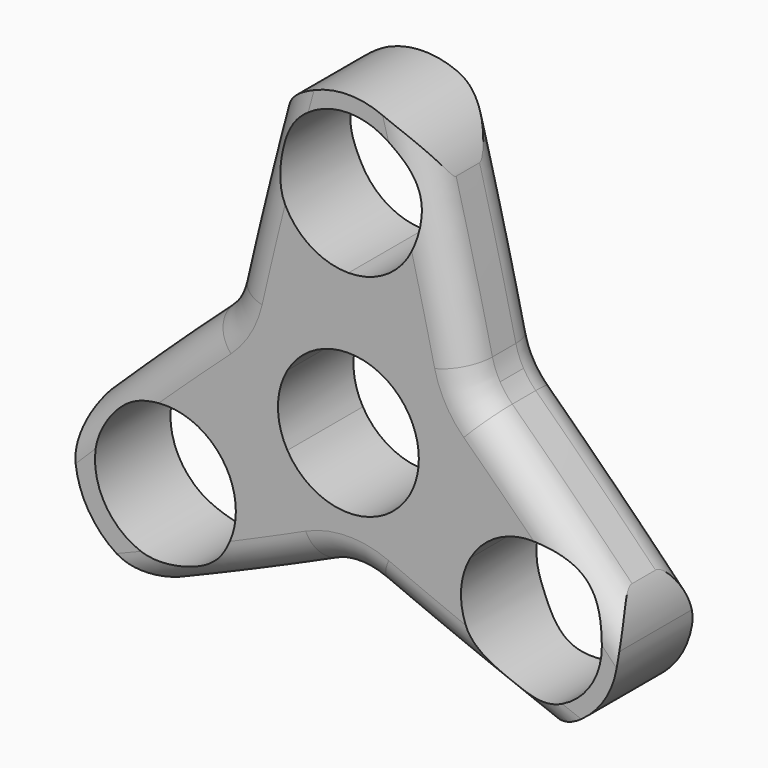
from build123d import *

# Parameters (mm, degrees)
F1_DEPTH     = 14.732
F2_T1_DEPTH  = 93.1608998229
F2_T3_DEPTH  = 105.6007192325
F2_T5_DEPTH  = 102.6342510382
F2_T7_DEPTH  = 101.1360229165
F2_T9_DEPTH  = 92.8404275057
F2_T11_DEPTH = 101.5905654736
F3_T3_ANGLE  = 47.4760223414
F3_T6_ANGLE  = 33.2408882111
F3_T9_ANGLE  = 34.8968457707
F3_T12_ANGLE = 2.7372148443
F3_T15_ANGLE = 2.8789593755
F3_T18_ANGLE = 2.9381084854
F3_T21_ANGLE = 2.7373414603
F3_T24_ANGLE = 2.9000589004
F3_T27_ANGLE = 2.9243217111
F4_T2_ANGLE  = 34.8968457707
F4_T4_ANGLE  = 33.2408882111
F4_T6_ANGLE  = 47.4760223414
F4_T8_ANGLE  = 2.9243217111
F4_T10_ANGLE = 2.9000589004
F4_T12_ANGLE = 2.8789593755
F4_T14_ANGLE = 2.7372148443
F4_T16_ANGLE = 2.7373414603
F4_T18_ANGLE = 2.9381084854


# Not quite as in the source:
# - a fillet or chamfer that OpenCascade refuses, or shapes differently, is made with other operations: its cross-section is extruded or revolved along the edge and cut away or added


with BuildPart() as f1:
    # F0 (on Front) → F1 (new body)
    with BuildSketch(Plane.XZ):
        with BuildLine():
            ThreePointArc((9.5262794416, 5.5), (10.6251840892, 2.8470094961), (11, 0))
            ThreePointArc((11, 0), (10.6251840892, -2.8470094961), (9.5262794416, -5.5))
            Line((9.5262794416, -5.5), (16.8874953738, -9.75))
            ThreePointArc((16.8874953738, -9.75), (28.5479373043, -3.0000353657), (40.239157826, -9.6965487338))
            Line((40.239157826, -9.6965487338), (31.0803296346, 6.00061125))
            ThreePointArc((31.0803296346, 6.00061125), (24.510706985, 6.8563515201), (19.6241089469, 11.3299845831))
            Line((19.6241089469, 11.3299845831), (9.5262794416, 5.5))
        make_face()
        with BuildLine():
            ThreePointArc((0, 11), (5.5, 9.5262794416), (9.5262794416, 5.5))
            Line((9.5262794416, 5.5), (19.6241089469, 11.3299845831))
            ThreePointArc((19.6241089469, 11.3299845831), (18.1888081178, 17.7485475745), (20.6723210956, 23.8387202021))
            Line((20.6723210956, 23.8387202021), (12.7673255725, 37.3869576844))
            ThreePointArc((12.7673255725, 37.3869576844), (13.3155716218, 35.2238597945), (13.5, 33))
            ThreePointArc((13.5, 33), (9.545941546, 23.454058454), (0, 19.5))
            Line((0, 19.5), (0, 11))
        make_face()
        with BuildLine():
            Line((16.8874953738, -9.75), (9.5262794416, -5.5))
            ThreePointArc((9.5262794416, -5.5), (0, -11), (-9.5262794416, -5.5))
            Line((-9.5262794416, -5.5), (-16.3617556921, -9.4464640532))
            ThreePointArc((-16.3617556921, -9.4464640532), (-14.9524532496, -12.8488211233), (-14.4717664314, -16.5))
            ThreePointArc((-14.4717664314, -16.5), (-18.4982539824, -26.3687028896), (-28.2792096, -30.6038895357))
            Line((-28.2792096, -30.6038895357), (-10.999379621, -30.4203603981))
            ThreePointArc((-10.999379621, -30.4203603981), (-0.1168244513, -19.3041563257), (10.999379621, -30.1867114954))
            Line((10.999379621, -30.1867114954), (28.5788383249, -30))
            ThreePointArc((28.5788383249, -30), (16.8874953738, -23.25), (16.8874953738, -9.75))
        make_face()
        with BuildLine():
            ThreePointArc((-9.5262794416, 5.5), (-5.5, 9.5262794416), (0, 11))
            Line((0, 11), (0, 19.5))
            ThreePointArc((0, 19.5), (-10.9880373302, 25.1569753519), (-12.7673255725, 37.3869576844))
            Line((-12.7673255725, 37.3869576844), (-20.7877581765, 23.9813723283))
            ThreePointArc((-20.7877581765, 23.9813723283), (-18.1883185789, 17.83960184), (-19.6151289856, 11.3248))
            Line((-19.6151289856, 11.3248), (-9.5262794416, 5.5))
        make_face()
        with BuildLine():
            Line((-16.3617556921, -9.4464640532), (-9.5262794416, -5.5))
            ThreePointArc((-9.5262794416, -5.5), (-11, 0), (-9.5262794416, 5.5))
            Line((-9.5262794416, 5.5), (-19.6151289856, 11.3248))
            ThreePointArc((-19.6151289856, 11.3248), (-24.6997770254, 6.7614054191), (-31.497874892, 6.080170374))
            Line((-31.497874892, 6.080170374), (-40.4168007072, -8.8271827831))
            ThreePointArc((-40.4168007072, -8.8271827831), (-28.2157813542, -2.3976006636), (-16.3617556921, -9.4464640532))
        make_face()
        with BuildLine():
            ThreePointArc((40.239157826, -9.6965487338), (28.5479373043, -3.0000353657), (16.8874953738, -9.75))
            ThreePointArc((16.8874953738, -9.75), (16.8874953738, -23.25), (28.5788383249, -30))
            ThreePointArc((28.5788383249, -30), (38.1247798709, -26.045941546), (42.0788383249, -16.5))
            ThreePointArc((42.0788383249, -16.5), (41.6108050465, -12.9761039506), (40.239157826, -9.6965487338))
        make_face()
        with BuildLine():
            ThreePointArc((39.5788383249, -16.5), (25.7318288288, -27.1251840892), (19.0525588833, -11))
            ThreePointArc((19.0525588833, -11), (31.425847821, -5.8748159108), (39.5788383249, -16.5))
        make_face(mode=Mode.SUBTRACT)
        with BuildLine():
            ThreePointArc((-12.7673255725, 37.3869576844), (-10.9880373302, 25.1569753519), (0, 19.5))
            ThreePointArc((0, 19.5), (9.545941546, 23.454058454), (13.5, 33))
            ThreePointArc((13.5, 33), (13.3155716218, 35.2238597945), (12.7673255725, 37.3869576844))
            ThreePointArc((12.7673255725, 37.3869576844), (0, 46.5), (-12.7673255725, 37.3869576844))
        make_face()
        with BuildLine():
            ThreePointArc((11, 33), (7.7781745931, 25.2218254069), (0, 22))
            ThreePointArc((0, 22), (-7.7781745931, 40.7781745931), (11, 33))
        make_face(mode=Mode.SUBTRACT)
        with BuildLine():
            ThreePointArc((-14.4717664314, -16.5), (-14.9524532496, -12.8488211233), (-16.3617556921, -9.4464640532))
            ThreePointArc((-16.3617556921, -9.4464640532), (-28.2157813542, -2.3976006636), (-40.4168007072, -8.8271827831))
            Line((-40.4168007072, -8.8271827831), (-40.9369339823, -9.6965487338))
            ThreePointArc((-40.9369339823, -9.6965487338), (-40.7235131568, -23.6774891596), (-28.5788383249, -30.6070718935))
            Line((-28.5788383249, -30.6070718935), (-28.2792096, -30.6038895357))
            ThreePointArc((-28.2792096, -30.6038895357), (-18.4982539824, -26.3687028896), (-14.4717664314, -16.5))
        make_face()
        with BuildLine():
            ThreePointArc((-17.5788383249, -16.5), (-39.2040224141, -19.3470094961), (-19.0525588833, -11))
            ThreePointArc((-19.0525588833, -11), (-17.9536542357, -13.6529905039), (-17.5788383249, -16.5))
        make_face(mode=Mode.SUBTRACT)
        with BuildLine():
            Line((-40.9369339823, -9.6965487338), (-40.4168007072, -8.8271827831))
            ThreePointArc((-40.4168007072, -8.8271827831), (-40.6846739199, -9.2571951597), (-40.9369339823, -9.6965487338))
        make_face()
        with BuildLine():
            ThreePointArc((-28.5788383249, -30.6070718935), (-28.4290155127, -30.6062762816), (-28.2792096, -30.6038895357))
            Line((-28.2792096, -30.6038895357), (-28.5788383249, -30.6070718935))
        make_face()
    extrude(amount=F1_DEPTH)

    # F2: fillet of radius 762 on 6 edges, made by hand

    # F2_s2 → F2_t1 (cut)
    with BuildSketch(Plane.XZ.offset(-39.2144499115)):
        with BuildLine():
            ThreePointArc((18.4292121278, 14.3690133138), (15.6877786705, 25.9000028626), (12.7673255725, 37.3869576844))
            Line((12.7673255725, 37.3869576844), (20.6723210956, 23.8387202021))
            ThreePointArc((20.6723210956, 23.8387202021), (18.4465771329, 19.3654183932), (18.4292121278, 14.3690133138))
        make_face()
    extrude(amount=F2_T1_DEPTH, mode=Mode.SUBTRACT)

    # F2_s4 → F2_t3 (cut)
    with BuildSketch(Plane.XZ.offset(-45.4343596162)):
        with BuildLine():
            ThreePointArc((40.239157826, -9.6965487338), (30.9662630608, -0.3199499106), (21.5324889533, 8.8947714041))
            ThreePointArc((21.5324889533, 8.8947714041), (25.9594233559, 6.302983958), (31.0803296346, 6.00061125))
            Line((31.0803296346, 6.00061125), (40.239157826, -9.6965487338))
        make_face()
    extrude(amount=F2_T3_DEPTH, mode=Mode.SUBTRACT)

    # F2_s6 → F2_t5 (cut)
    with BuildSketch(Plane.XZ.offset(-43.9511255191)):
        with BuildLine():
            ThreePointArc((4.299605952, -20.178646384), (16.3970231968, -25.1936426117), (28.5788383249, -30))
            Line((28.5788383249, -30), (10.999379621, -30.1867114954))
            ThreePointArc((10.999379621, -30.1867114954), (9.1408468814, -24.1843106453), (4.299605952, -20.178646384))
        make_face()
    extrude(amount=F2_T5_DEPTH, mode=Mode.SUBTRACT)

    # F2_s8 → F2_t7 (cut)
    with BuildSketch(Plane.XZ.offset(-43.2020114583)):
        with BuildLine():
            ThreePointArc((-28.2792096, -30.6038895357), (-16.3737864916, -25.5482948848), (-4.5558903431, -20.2913502123))
            ThreePointArc((-4.5558903431, -20.2913502123), (-9.2812077743, -24.3993694307), (-10.999379621, -30.4203603981))
            Line((-10.999379621, -30.4203603981), (-28.2792096, -30.6038895357))
        make_face()
    extrude(amount=F2_T7_DEPTH, mode=Mode.SUBTRACT)

    # F2_s10 → F2_t9 (cut)
    with BuildSketch(Plane.XZ.offset(-39.0542137528)):
        with BuildLine():
            ThreePointArc((-12.7673255725, 37.3869576844), (-15.6827737348, 25.899600201), (-18.4192093403, 14.3682889089))
            ThreePointArc((-18.4192093403, 14.3682889089), (-18.4608255688, 19.4563679368), (-20.7877581765, 23.9813723283))
            Line((-20.7877581765, 23.9813723283), (-12.7673255725, 37.3869576844))
        make_face()
    extrude(amount=F2_T9_DEPTH, mode=Mode.SUBTRACT)

    # F2_s12 → F2_t11 (cut)
    with BuildSketch(Plane.XZ.offset(-43.4292827368)):
        with BuildLine():
            ThreePointArc((-21.7526107908, 8.6758326121), (-31.1581778052, 0.0026712097), (-40.4168007072, -8.8271827831))
            Line((-40.4168007072, -8.8271827831), (-31.497874892, 6.080170374))
            ThreePointArc((-31.497874892, 6.080170374), (-26.3102505601, 6.195381148), (-21.7526107908, 8.6758326121))
        make_face()
    extrude(amount=F2_T11_DEPTH, mode=Mode.SUBTRACT)

    # F3: fillet of radius 5.08 on 3 edges, made by hand


with BuildPart() as f3_tool1:
    # F3_s2 → F3_t3 (revolve)
    with BuildSketch(Plane(origin=(-11.4237869858, 0, -5.198217671), x_dir=(0, 1, 0), z_dir=(-0.9101987031, 0, -0.4141718494))):
        with BuildLine():
            ThreePointArc((-14.732, 11.5022391191), (-13.2441024484, 15.0943415675), (-9.652, 16.5822391191))
            Line((-9.652, 16.5822391191), (-14.732, 16.5822391191))
            Line((-14.732, 16.5822391191), (-14.732, 11.5022391191))
        make_face()
    revolve(axis=Axis((0, -14.732, -30.3035359468), (0, 1, 0)), revolution_arc=F3_T3_ANGLE)


with BuildPart() as f3_tool4:
    # F3_s5 → F3_t6 (revolve)
    with BuildSketch(Plane(origin=(6.7616814576, 0, -6.4912949652), x_dir=(0, 1, 0), z_dir=(0.7213830163, 0, -0.6925363123))):
        with BuildLine():
            ThreePointArc((-14.732, 16.2485675186), (-13.2441024484, 19.8406699671), (-9.652, 21.3285675186))
            Line((-9.652, 21.3285675186), (-14.732, 21.3285675186))
            Line((-14.732, 21.3285675186), (-14.732, 16.2485675186))
        make_face()
    revolve(axis=Axis((29.1503883885, -14.732, 16.8299845831), (0, 1, 0)), revolution_arc=F3_T6_ANGLE)


with BuildPart() as f3_tool7:
    # F3_s8 → F3_t9 (revolve)
    with BuildSketch(Plane(origin=(2.209086872, 0, 9.6422398936), x_dir=(0, 1, 0), z_dir=(0.2233191901, 0, 0.9747453715))):
        with BuildLine():
            ThreePointArc((-14.732, 16.0827536941), (-13.2441024484, 19.6748561425), (-9.652, 21.1627536941))
            Line((-9.652, 21.1627536941), (-14.732, 21.1627536941))
            Line((-14.732, 21.1627536941), (-14.732, 16.0827536941))
        make_face()
    revolve(axis=Axis((-29.1414084272, -14.732, 16.8248), (0, 1, 0)), revolution_arc=F3_T9_ANGLE)


with BuildPart() as f3_tool10:
    # F3_s11 → F3_t12 (revolve)
    with BuildSketch(Plane(origin=(2.209086872, 0, 9.6422398938), x_dir=(0, 1, 0), z_dir=(-0.2233191901, 0, -0.9747453715))):
        with BuildLine():
            ThreePointArc((-14.732, -16.082753694), (-13.2441024484, -19.6748561424), (-9.652, -21.162753694))
            Line((-9.652, -21.162753694), (-14.732, -21.162753694))
            Line((-14.732, -21.162753694), (-14.732, -16.082753694))
        make_face()
    revolve(axis=Axis((724.3367633965, -14.732, -155.800933855), (0, 1, 0)), revolution_arc=F3_T12_ANGLE)


with BuildPart() as f3_tool13:
    # F3_s14 → F3_t15 (revolve)
    with BuildSketch(Plane(origin=(-33.5345165919, 0, -33.6260087343), x_dir=(0, 1, 0), z_dir=(-0.7061428411, 0, -0.708069409))):
        with BuildLine():
            ThreePointArc((-14.732, -17.4104791821), (-13.2441024484, -21.0025816305), (-9.652, -22.4904791821))
            Line((-9.652, -22.4904791821), (-14.732, -22.4904791821))
            Line((-14.732, -22.4904791821), (-14.732, -17.4104791821))
        make_face()
    revolve(axis=Axis((490.0895527499, -14.732, -555.8253628125), (0, 1, 0)), revolution_arc=F3_T15_ANGLE)


with BuildPart() as f3_tool16:
    # F3_s17 → F3_t18 (revolve)
    with BuildSketch(Plane(origin=(6.7616814574, 0, -6.4912949651), x_dir=(0, 1, 0), z_dir=(-0.7213830163, 0, 0.6925363123))):
        with BuildLine():
            ThreePointArc((-9.652, -21.3285675187), (-13.2441024484, -19.8406699671), (-14.732, -16.2485675187))
            Line((-14.732, -16.2485675187), (-14.732, -21.3285675187))
            Line((-14.732, -21.3285675187), (-9.652, -21.3285675187))
        make_face()
    revolve(axis=Axis((-506.1801812267, -14.732, -540.7990872124), (0, 1, 0)), revolution_arc=F3_T18_ANGLE)


with BuildPart() as f3_tool19:
    # F3_s20 → F3_t21 (revolve)
    with BuildSketch(Plane(origin=(-12.2183116584, 0, 43.5694879997), x_dir=(0, 1, 0), z_dir=(-0.2700162938, 0, 0.962855753))):
        with BuildLine():
            ThreePointArc((-14.732, -17.4140115449), (-13.2441024484, -21.0061139934), (-9.652, -22.4940115449))
            Line((-9.652, -22.4940115449), (-14.732, -22.4940115449))
            Line((-14.732, -22.4940115449), (-14.732, -17.4140115449))
        make_face()
    revolve(axis=Axis((-724.2559071439, -14.732, -156.1091782762), (0, 1, 0)), revolution_arc=F3_T21_ANGLE)


with BuildPart() as f3_tool22:
    # F3_s23 → F3_t24 (revolve)
    with BuildSketch(Plane(origin=(-11.4237869859, 0, -5.1982176711), x_dir=(0, 1, 0), z_dir=(0.9101987031, 0, 0.4141718494))):
        with BuildLine():
            ThreePointArc((-14.732, -11.502239119), (-13.2441024484, -15.0943415675), (-9.652, -16.582239119))
            Line((-9.652, -16.582239119), (-14.732, -16.582239119))
            Line((-14.732, -16.582239119), (-14.732, -11.502239119))
        make_face()
    revolve(axis=Axis((-320.1548394701, -14.732, 673.2800613529), (0, 1, 0)), revolution_arc=F3_T24_ANGLE)


with BuildPart() as f3_tool25:
    # F3_s26 → F3_t27 (revolve)
    with BuildSketch(Plane(origin=(46.811401932, 0, -17.1162062944), x_dir=(0, 1, 0), z_dir=(0.9391870313, 0, -0.3434060574))):
        with BuildLine():
            ThreePointArc((-9.652, -18.4672956703), (-13.2441024484, -16.9793981188), (-14.732, -13.3872956703))
            Line((-14.732, -13.3872956703), (-14.732, -18.4672956703))
            Line((-14.732, -18.4672956703), (-9.652, -18.4672956703))
        make_face()
    revolve(axis=Axis((302.1450363799, -14.732, 681.2000667914), (0, 1, 0)), revolution_arc=F3_T27_ANGLE)


with BuildPart() as f1_1:
    add(f1.part)

    # F3_t28: cut F3_tool1, F3_tool4, F3_tool7, F3_tool10, F3_tool13, F3_tool16, F3_tool19, F3_tool22, F3_tool25
    add([f3_tool1.part, f3_tool4.part, f3_tool7.part, f3_tool10.part, f3_tool13.part, f3_tool16.part, f3_tool19.part, f3_tool22.part, f3_tool25.part], mode=Mode.SUBTRACT)

    # F4: fillet of radius 5.08 on 9 edges, made by hand

    # F4_s1 → F4_t2 (revolve, cut)
    with BuildSketch(Plane(origin=(2.209086872, 0, 9.6422398936), x_dir=(0, 1, 0), z_dir=(0.2233191901, 0, 0.9747453715))):
        with BuildLine():
            ThreePointArc((0, 16.0827536941), (-1.4878975516, 19.6748561425), (-5.08, 21.1627536941))
            Line((-5.08, 21.1627536941), (0, 21.1627536941))
            Line((0, 21.1627536941), (0, 16.0827536941))
        make_face()
    revolve(axis=Axis((-29.1414084272, 0, 16.8248), (0, 1, 0)), revolution_arc=F4_T2_ANGLE, mode=Mode.SUBTRACT)

    # F4_s3 → F4_t4 (revolve, cut)
    with BuildSketch(Plane(origin=(6.7616814576, 0, -6.4912949652), x_dir=(0, 1, 0), z_dir=(0.7213830163, 0, -0.6925363123))):
        with BuildLine():
            ThreePointArc((0, 16.2485675186), (-1.4878975516, 19.8406699671), (-5.08, 21.3285675186))
            Line((-5.08, 21.3285675186), (0, 21.3285675186))
            Line((0, 21.3285675186), (0, 16.2485675186))
        make_face()
    revolve(axis=Axis((29.1503883885, 0, 16.8299845831), (0, 1, 0)), revolution_arc=F4_T4_ANGLE, mode=Mode.SUBTRACT)

    # F4_s5 → F4_t6 (revolve, cut)
    with BuildSketch(Plane(origin=(-11.4237869858, 0, -5.198217671), x_dir=(0, 1, 0), z_dir=(-0.9101987031, 0, -0.4141718494))):
        with BuildLine():
            ThreePointArc((0, 11.5022391191), (-1.4878975516, 15.0943415675), (-5.08, 16.5822391191))
            Line((-5.08, 16.5822391191), (0, 16.5822391191))
            Line((0, 16.5822391191), (0, 11.5022391191))
        make_face()
    revolve(axis=Axis((0, 0, -30.3035359468), (0, 1, 0)), revolution_arc=F4_T6_ANGLE, mode=Mode.SUBTRACT)

    # F4_s7 → F4_t8 (revolve, cut)
    with BuildSketch(Plane(origin=(46.811401932, 0, -17.1162062944), x_dir=(0, 1, 0), z_dir=(0.9391870313, 0, -0.3434060574))):
        with BuildLine():
            ThreePointArc((0, -13.3872956703), (-1.4878975516, -16.9793981188), (-5.08, -18.4672956703))
            Line((-5.08, -18.4672956703), (0, -18.4672956703))
            Line((0, -18.4672956703), (0, -13.3872956703))
        make_face()
    revolve(axis=Axis((302.1450363799, 0, 681.2000667914), (0, 1, 0)), revolution_arc=F4_T8_ANGLE, mode=Mode.SUBTRACT)

    # F4_s9 → F4_t10 (revolve, cut)
    with BuildSketch(Plane(origin=(-11.4237869859, 0, -5.1982176711), x_dir=(0, 1, 0), z_dir=(0.9101987031, 0, 0.4141718494))):
        with BuildLine():
            ThreePointArc((0, -11.502239119), (-1.4878975516, -15.0943415675), (-5.08, -16.582239119))
            Line((-5.08, -16.582239119), (0, -16.582239119))
            Line((0, -16.582239119), (0, -11.502239119))
        make_face()
    revolve(axis=Axis((-320.1548394701, 0, 673.2800613529), (0, 1, 0)), revolution_arc=F4_T10_ANGLE, mode=Mode.SUBTRACT)

    # F4_s11 → F4_t12 (revolve, cut)
    with BuildSketch(Plane(origin=(-33.5345165919, 0, -33.6260087343), x_dir=(0, 1, 0), z_dir=(-0.7061428411, 0, -0.708069409))):
        with BuildLine():
            ThreePointArc((0, -17.4104791821), (-1.4878975516, -21.0025816305), (-5.08, -22.4904791821))
            Line((-5.08, -22.4904791821), (0, -22.4904791821))
            Line((0, -22.4904791821), (0, -17.4104791821))
        make_face()
    revolve(axis=Axis((490.0895527499, 0, -555.8253628125), (0, 1, 0)), revolution_arc=F4_T12_ANGLE, mode=Mode.SUBTRACT)

    # F4_s13 → F4_t14 (revolve, cut)
    with BuildSketch(Plane(origin=(2.209086872, 0, 9.6422398938), x_dir=(0, 1, 0), z_dir=(-0.2233191901, 0, -0.9747453715))):
        with BuildLine():
            ThreePointArc((0, -16.082753694), (-1.4878975516, -19.6748561424), (-5.08, -21.162753694))
            Line((-5.08, -21.162753694), (0, -21.162753694))
            Line((0, -21.162753694), (0, -16.082753694))
        make_face()
    revolve(axis=Axis((724.3367633965, 0, -155.800933855), (0, 1, 0)), revolution_arc=F4_T14_ANGLE, mode=Mode.SUBTRACT)

    # F4_s15 → F4_t16 (revolve, cut)
    with BuildSketch(Plane(origin=(-12.2183116584, 0, 43.5694879997), x_dir=(0, 1, 0), z_dir=(-0.2700162938, 0, 0.962855753))):
        with BuildLine():
            ThreePointArc((0, -17.4140115449), (-1.4878975516, -21.0061139934), (-5.08, -22.4940115449))
            Line((-5.08, -22.4940115449), (0, -22.4940115449))
            Line((0, -22.4940115449), (0, -17.4140115449))
        make_face()
    revolve(axis=Axis((-724.2559071439, 0, -156.1091782762), (0, 1, 0)), revolution_arc=F4_T16_ANGLE, mode=Mode.SUBTRACT)

    # F4_s17 → F4_t18 (revolve, cut)
    with BuildSketch(Plane(origin=(6.7616814574, 0, -6.4912949651), x_dir=(0, 1, 0), z_dir=(-0.7213830163, 0, 0.6925363123))):
        with BuildLine():
            ThreePointArc((0, -16.2485675187), (-1.4878975516, -19.8406699671), (-5.08, -21.3285675187))
            Line((-5.08, -21.3285675187), (0, -21.3285675187))
            Line((0, -21.3285675187), (0, -16.2485675187))
        make_face()
    revolve(axis=Axis((-506.1801812267, 0, -540.7990872124), (0, 1, 0)), revolution_arc=F4_T18_ANGLE, mode=Mode.SUBTRACT)


solid = f1_1.part
